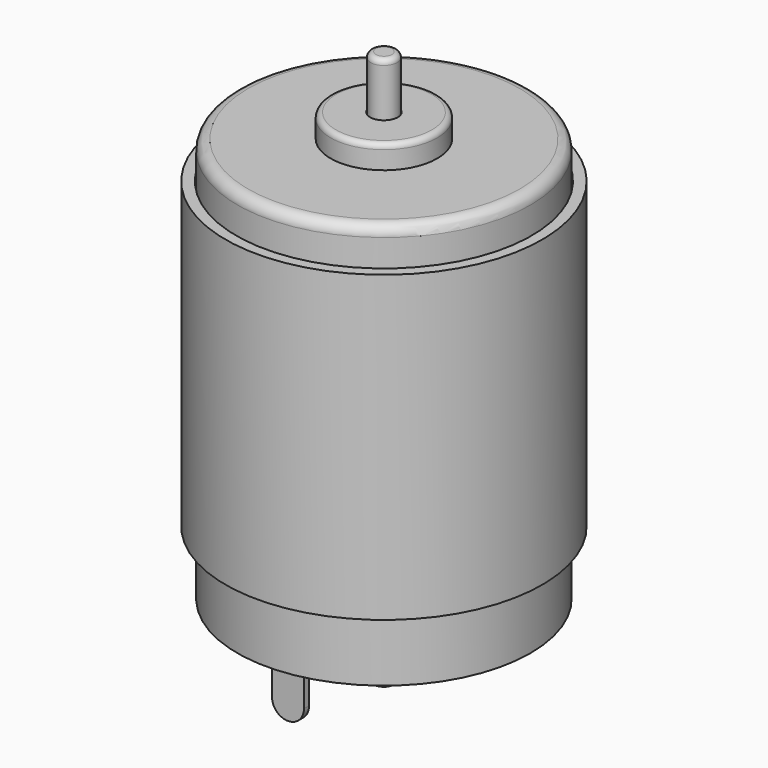
from build123d import *

# Parameters (mm, degrees)
F0_R           = 13.75
F1_DEPTH       = 38
F2_R           = 5
F3_DEPTH       = 2.2
F4_R           = 1
F5_R           = 0.5
F6_R           = 4.95
F7_DEPTH       = 2.5
F8_R           = 3.225
F9_DEPTH       = 0.9
F9_TAPER       = 5
F10_R          = 2.6462602028
F11_DEPTH      = 1.2
F12_R          = 1.3
F13_DEPTH      = 42.401
F14_R          = 1.25
F15_DEPTH      = 5
F15_DEPTH_BACK = 47
F16_R          = 0.5
F17_R          = 0.5
F18_W          = 3
F18_H          = 0.6
F19_DEPTH      = 5.5
F20_R          = 1.49999
F21_R          = 14.85
F21_R_2        = 13.85
F22_DEPTH      = 34.5
F23_DEPTH      = 6
F24_W          = 6.5
F24_H          = 28.5
F25_DEPTH      = 25


# Not quite as in the source:
# - a fillet or chamfer is up to 0.001 mm smaller than in the source, because OpenCascade refuses the exact size


with BuildPart() as f1:
    # F0 (on Top) → F1 (new body)
    with BuildSketch(Plane.XY):
        Circle(F0_R)
    extrude(amount=F1_DEPTH)

    # F2 (on face) → F3 (join)
    with BuildSketch(Plane.XY.offset(38)):
        Circle(F2_R)
    extrude(amount=F3_DEPTH)

    # F4
    f4_edges = [f1.edges().sort_by_distance(p)[0] for p in [
        (-13.75, 0, 38),
    ]]
    fillet(f4_edges, radius=F4_R)

    # F5
    f5_edges = [f1.edges().sort_by_distance(p)[0] for p in [
        (-5, 0, 40.2),
    ]]
    fillet(f5_edges, radius=F5_R)

    # F6 (on face) → F7 (join)
    with BuildSketch(Plane(origin=(0, 0, 0), x_dir=(1, 0, 0), z_dir=(0, 0, -1))):
        Circle(F6_R)
    extrude(amount=F7_DEPTH)

    # F8 (on face) → F9 (join)
    with BuildSketch(Plane(origin=(0, 0, -2.5), x_dir=(1, 0, 0), z_dir=(0, 0, -1))):
        Circle(F8_R)
    extrude(amount=F9_DEPTH, taper=F9_TAPER)

    # F10 (on face) → F11 (cut)
    with BuildSketch(Plane(origin=(0, 0, -3.4), x_dir=(1, 0, 0), z_dir=(0, 0, -1))):
        Circle(F10_R)
    extrude(amount=-F11_DEPTH, mode=Mode.SUBTRACT)

    # F12 (on face) → F13 (cut, through all)
    with BuildSketch(Plane(origin=(0, 0, -2.2), x_dir=(1, 0, 0), z_dir=(0, 0, -1))):
        Circle(F12_R)
    extrude(amount=-F13_DEPTH, mode=Mode.SUBTRACT)

    # F18 (on face) → F19 (join)
    with BuildSketch(Plane(origin=(0, 0, 0), x_dir=(1, 0, 0), z_dir=(0, 0, -1))):
        with Locations((0, -10.95)):
            Rectangle(F18_W, F18_H)
        with Locations((0, 10.95)):
            Rectangle(F18_W, F18_H)
    extrude(amount=F19_DEPTH)

    # F20 (radius 1.5 in the source; OpenCascade refuses exactly that, so slightly less here)
    f20_edges = [f1.edges().sort_by_distance(p)[0] for p in [
        (1.5, 10.95, -5.5),
        (-1.5, 10.95, -5.5),
        (1.5, -10.95, -5.5),
        (-1.5, -10.95, -5.5),
    ]]
    fillet(f20_edges, radius=F20_R)


with BuildPart() as f15:
    # F14 (on face) → F15 (new body, two sides)
    with BuildSketch(Plane.XY.offset(40.2)) as f15_sk:
        Circle(F14_R)
    extrude(amount=F15_DEPTH)
    extrude(f15_sk.sketch, amount=-F15_DEPTH_BACK)

    # F16
    f16_edges = [f15.edges().sort_by_distance(p)[0] for p in [
        (-1.25, 0, 45.2),
    ]]
    fillet(f16_edges, radius=F16_R)

    # F17
    f17_edges = [f15.edges().sort_by_distance(p)[0] for p in [
        (-1.25, 0, -6.8),
    ]]
    fillet(f17_edges, radius=F17_R)


with BuildPart() as f22:
    # F21 (on Top) → F22 (new body)
    with BuildSketch(Plane.XY):
        Circle(F21_R)
        Circle(F21_R_2, mode=Mode.SUBTRACT)
    extrude(amount=F22_DEPTH)

    # F23 (cut): a face of the model
    f23_faces = [f22.faces().sort_by_distance(p)[0] for p in [
        (-14.429978572, 0, 0),
    ]]
    extrude(f23_faces, amount=-F23_DEPTH, mode=Mode.SUBTRACT)

    # F24 (on Front) → F25 (cut)
    with BuildSketch(Plane.XZ):
        with Locations((0, 20.25)):
            Rectangle(F24_W, F24_H)
    extrude(amount=-F25_DEPTH, mode=Mode.SUBTRACT)


solid = Compound([f1.part, f15.part, f22.part])
